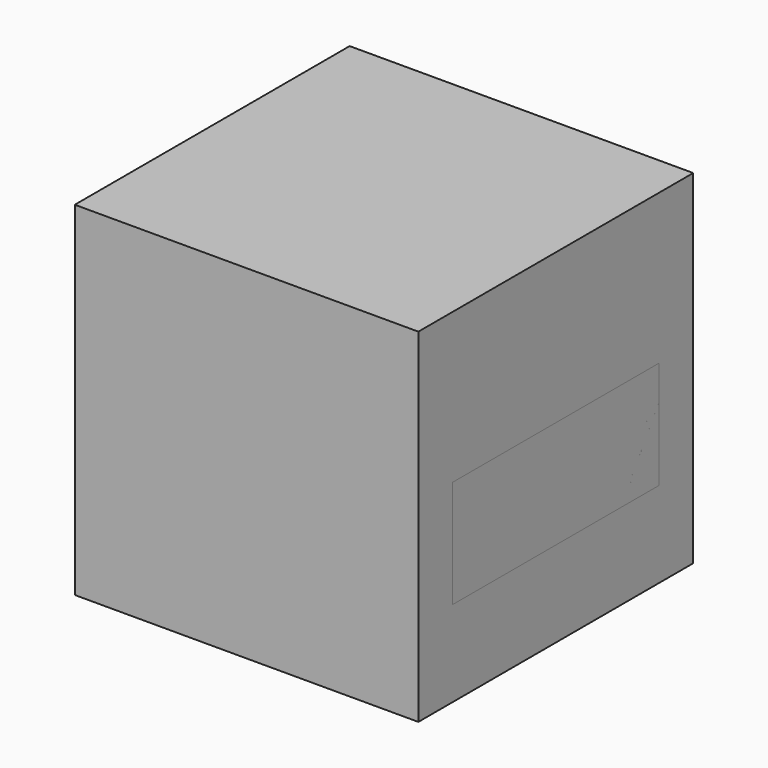
from build123d import *

# Parameters (mm, degrees)
F0_W     = 101.6
F0_H     = 101.6
F1_DEPTH = 50.8
F2_W     = 76.2
F2_H     = 50.8
F3_DEPTH = 50.8
F4_W     = 87.0356416881
F4_H     = 18.9636399314
F5_DEPTH = 135.89
F6_R     = 3
F6_R_2   = 2.9972
F7_DEPTH = 25.4


with BuildPart() as f1:
    # F0 (on Front) → F1 (new body, symmetric)
    with BuildSketch(Plane.XZ):
        Rectangle(F0_W, F0_H)
    extrude(amount=F1_DEPTH, both=True)


with BuildPart() as f3:
    # F2 (on Right) → F3 (new body, symmetric)
    with BuildSketch(Plane.YZ):
        Rectangle(F2_W, F2_H)
    extrude(amount=F3_DEPTH, both=True)

    # F4 (on face) → F5 (cut)
    with BuildSketch(Plane(origin=(0, 38.1, 0), x_dir=(-1, 0, 0), z_dir=(0, 1, 0))):
        with Locations((-7.2821791559, 15.9181800343)):
            Rectangle(F4_W, F4_H)
    extrude(amount=-F5_DEPTH, mode=Mode.SUBTRACT)

    # F6 (on face) → F7 (cut)
    with BuildSketch(Plane.XY.offset(6.4363600686)):
        with Locations((-27.9406899035, 25.62)):
            Circle(F6_R)
        with Locations((-19.2760222971, 25.62)):
            Circle(F6_R)
        with Locations((-27.9406899035, 17.08)):
            Circle(F6_R)
        with Locations((-19.2760222971, 17.08)):
            Circle(F6_R)
        with Locations((-27.9406899035, 8.54)):
            Circle(F6_R)
        with Locations((-19.2760222971, 8.54)):
            Circle(F6_R)
        with BuildLine():
            ThreePointArc((-24.9406899035, 0), (-27.9406899035, 3), (-30.9406899035, 0))
            Line((-30.9406899035, 0), (-24.9406899035, 0))
        make_face()
        with BuildLine():
            ThreePointArc((-22.2760222971, 0), (-19.2760222971, -3), (-16.2760222971, 0))
            Line((-16.2760222971, 0), (-22.2760222971, 0))
        make_face()
        with BuildLine():
            Line((-22.2760222971, 0), (-16.2760222971, 0))
            ThreePointArc((-16.2760222971, 0), (-19.2760222971, 3), (-22.2760222971, 0))
        make_face()
        with BuildLine():
            Line((-24.9406899035, 0), (-30.9406899035, 0))
            ThreePointArc((-30.9406899035, 0), (-27.9406899035, -3), (-24.9406899035, 0))
        make_face()
        with Locations((-27.9406899035, -8.54)):
            Circle(F6_R)
        with Locations((-19.2760222971, -8.54)):
            Circle(F6_R)
        with Locations((-19.2760222971, -17.08)):
            Circle(F6_R)
        with Locations((-27.9406899035, -25.62)):
            Circle(F6_R)
        with Locations((-19.2760222971, -25.62)):
            Circle(F6_R)
        with Locations((-27.9406899035, -17.08)):
            Circle(F6_R)
        with BuildLine():
            ThreePointArc((33.840380609, 14.08), (31.194793451, 15.6654793784), (31.3455555481, 18.7460876073))
            ThreePointArc((31.3455555481, 18.7460876073), (20.0532603986, 24.7179373128), (7.2821791559, 24.4379327777))
            Line((7.2821791559, 24.4379327777), (7.2821791559, 0))
            Line((7.2821791559, 0), (30.840380609, 0))
            ThreePointArc((30.840380609, 0), (31.7190602655, 2.1213203436), (33.840380609, 3))
            Line((33.840380609, 3), (33.840380609, 5.54))
            ThreePointArc((33.840380609, 5.54), (30.840380609, 8.54), (33.840380609, 11.54))
            Line((33.840380609, 11.54), (33.840380609, 14.08))
        make_face()
        with BuildLine():
            Line((30.840380609, 0), (7.2821791559, 0))
            Line((7.2821791559, 0), (7.2821791559, -24.4379327777))
            ThreePointArc((7.2821791559, -24.4379327777), (20.0532603986, -24.7179373128), (31.3455555481, -18.7460876073))
            ThreePointArc((31.3455555481, -18.7460876073), (31.194793451, -15.6654793784), (33.840380609, -14.08))
            Line((33.840380609, -14.08), (33.840380609, -11.54))
            ThreePointArc((33.840380609, -11.54), (30.840380609, -8.54), (33.840380609, -5.54))
            Line((33.840380609, -5.54), (33.840380609, -3))
            ThreePointArc((33.840380609, -3), (31.7190602655, -2.1213203436), (30.840380609, 0))
        make_face()
        with BuildLine():
            Line((7.2821791559, -24.4379327777), (7.2821791559, 0))
            Line((7.2821791559, 0), (-11.1934117317, 0))
            ThreePointArc((-11.1934117317, 0), (-6.0547047735, -15.3179634506), (7.2821791559, -24.4379327777))
        make_face()
        with BuildLine():
            Line((7.2821791559, 0), (7.2821791559, 24.4379327777))
            ThreePointArc((7.2821791559, 24.4379327777), (-6.0547047735, 15.3179634506), (-11.1934117317, 0))
            Line((-11.1934117317, 0), (7.2821791559, 0))
        make_face()
        with BuildLine():
            ThreePointArc((38.1727144122, 8.4133701721), (36.8561037173, 11.4960623661), (35.1450168327, 14.3785329312))
            ThreePointArc((35.1450168327, 14.3785329312), (34.5095587593, 14.1555854256), (33.840380609, 14.08))
            Line((33.840380609, 14.08), (33.840380609, 11.54))
            ThreePointArc((33.840380609, 11.54), (35.9617009526, 10.6613203436), (36.840380609, 8.54))
            ThreePointArc((36.840380609, 8.54), (35.9617009526, 6.4186796564), (33.840380609, 5.54))
            Line((33.840380609, 5.54), (33.840380609, 3))
            ThreePointArc((33.840380609, 3), (35.9617009526, 2.1213203436), (36.840380609, 0))
            Line((36.840380609, 0), (38.1727144122, 0))
            Line((38.1727144122, 0), (38.1727144122, 8.4133701721))
        make_face()
        with BuildLine():
            Line((38.1727144122, -8.4133701721), (38.1727144122, 0))
            Line((38.1727144122, 0), (36.840380609, 0))
            ThreePointArc((36.840380609, 0), (35.9617009526, -2.1213203436), (33.840380609, -3))
            Line((33.840380609, -3), (33.840380609, -5.54))
            ThreePointArc((33.840380609, -5.54), (35.9617009526, -6.4186796564), (36.840380609, -8.54))
            ThreePointArc((36.840380609, -8.54), (35.9617009526, -10.6613203436), (33.840380609, -11.54))
            Line((33.840380609, -11.54), (33.840380609, -14.08))
            ThreePointArc((33.840380609, -14.08), (34.5095587593, -14.1555854256), (35.1450168327, -14.3785329312))
            ThreePointArc((35.1450168327, -14.3785329312), (36.8561037173, -11.4960623661), (38.1727144122, -8.4133701721))
        make_face()
        with BuildLine():
            Line((39.5050482154, 0), (38.1727144122, 0))
            Line((38.1727144122, 0), (38.1727144122, -8.4133701721))
            ThreePointArc((38.1727144122, -8.4133701721), (39.1813548402, -4.6282863649), (39.5960058914, -0.7331253354))
            ThreePointArc((39.5960058914, -0.7331253354), (39.5278744741, -0.3693731366), (39.5050482154, 0))
        make_face()
        with BuildLine():
            ThreePointArc((39.5960058914, 0.7331253354), (39.1813548402, 4.6282863649), (38.1727144122, 8.4133701721))
            Line((38.1727144122, 8.4133701721), (38.1727144122, 0))
            Line((38.1727144122, 0), (39.5050482154, 0))
            ThreePointArc((39.5050482154, 0), (39.5278744741, 0.3693731366), (39.5960058914, 0.7331253354))
        make_face()
        with BuildLine():
            ThreePointArc((33.840380609, 16.1144096485), (32.6399925862, 17.4748277603), (31.3455555481, 18.7460876073))
            ThreePointArc((31.3455555481, 18.7460876073), (31.194793451, 15.6654793784), (33.840380609, 14.08))
            Line((33.840380609, 14.08), (33.840380609, 16.1144096485))
        make_face()
        with BuildLine():
            ThreePointArc((33.840380609, -14.08), (31.194793451, -15.6654793784), (31.3455555481, -18.7460876073))
            ThreePointArc((31.3455555481, -18.7460876073), (32.6399925862, -17.4748277603), (33.840380609, -16.1144096485))
            Line((33.840380609, -16.1144096485), (33.840380609, -14.08))
        make_face()
        with BuildLine():
            Line((33.840380609, -11.54), (33.840380609, -5.54))
            ThreePointArc((33.840380609, -5.54), (30.840380609, -8.54), (33.840380609, -11.54))
        make_face()
        with BuildLine():
            ThreePointArc((36.840380609, -8.54), (35.9617009526, -6.4186796564), (33.840380609, -5.54))
            Line((33.840380609, -5.54), (33.840380609, -11.54))
            ThreePointArc((33.840380609, -11.54), (35.9617009526, -10.6613203436), (36.840380609, -8.54))
        make_face()
        with BuildLine():
            ThreePointArc((33.840380609, 3), (31.7190602655, 2.1213203436), (30.840380609, 0))
            Line((30.840380609, 0), (33.840380609, 0))
            Line((33.840380609, 0), (33.840380609, 3))
        make_face()
        with BuildLine():
            Line((33.840380609, 0), (30.840380609, 0))
            ThreePointArc((30.840380609, 0), (31.7190602655, -2.1213203436), (33.840380609, -3))
            Line((33.840380609, -3), (33.840380609, 0))
        make_face()
        with BuildLine():
            ThreePointArc((33.840380609, -3), (35.9617009526, -2.1213203436), (36.840380609, 0))
            Line((36.840380609, 0), (33.840380609, 0))
            Line((33.840380609, 0), (33.840380609, -3))
        make_face()
        with BuildLine():
            ThreePointArc((36.840380609, 8.54), (35.9617009526, 10.6613203436), (33.840380609, 11.54))
            Line((33.840380609, 11.54), (33.840380609, 5.54))
            ThreePointArc((33.840380609, 5.54), (35.9617009526, 6.4186796564), (36.840380609, 8.54))
        make_face()
        with BuildLine():
            Line((33.840380609, 5.54), (33.840380609, 11.54))
            ThreePointArc((33.840380609, 11.54), (30.840380609, 8.54), (33.840380609, 5.54))
        make_face()
        with BuildLine():
            Line((33.840380609, 0), (36.840380609, 0))
            ThreePointArc((36.840380609, 0), (35.9617009526, 2.1213203436), (33.840380609, 3))
            Line((33.840380609, 3), (33.840380609, 0))
        make_face()
        with BuildLine():
            ThreePointArc((33.840380609, -16.1144096485), (34.5112575414, -15.2604195785), (35.1450168327, -14.3785329312))
            ThreePointArc((35.1450168327, -14.3785329312), (34.5095587593, -14.1555854256), (33.840380609, -14.08))
            Line((33.840380609, -14.08), (33.840380609, -16.1144096485))
        make_face()
        with BuildLine():
            ThreePointArc((35.1450168327, 14.3785329312), (34.5112575414, 15.2604195785), (33.840380609, 16.1144096485))
            Line((33.840380609, 16.1144096485), (33.840380609, 14.08))
            ThreePointArc((33.840380609, 14.08), (34.5095587593, 14.1555854256), (35.1450168327, 14.3785329312))
        make_face()
        with BuildLine():
            Line((39.6065882683, 0), (39.5050482154, 0))
            ThreePointArc((39.5050482154, 0), (39.5278744741, -0.3693731366), (39.5960058914, -0.7331253354))
            ThreePointArc((39.5960058914, -0.7331253354), (39.6039425363, -0.3666008538), (39.6065882683, 0))
        make_face()
        with BuildLine():
            ThreePointArc((39.6065882683, 0), (39.6039425363, 0.3666008538), (39.5960058914, 0.7331253354))
            ThreePointArc((39.5960058914, 0.7331253354), (39.5278744741, 0.3693731366), (39.5050482154, 0))
            Line((39.5050482154, 0), (39.6065882683, 0))
        make_face()
        with Locations((-27.9406899035, 34.1572)):
            Circle(F6_R_2)
        with Locations((-19.2760222971, 34.1572)):
            Circle(F6_R_2)
        with Locations((-27.9406899035, -34.1572)):
            Circle(F6_R_2)
        with Locations((-19.2760222971, -34.1572)):
            Circle(F6_R_2)
    extrude(amount=-F7_DEPTH, mode=Mode.SUBTRACT)


solid = Compound([f1.part, f3.part])
